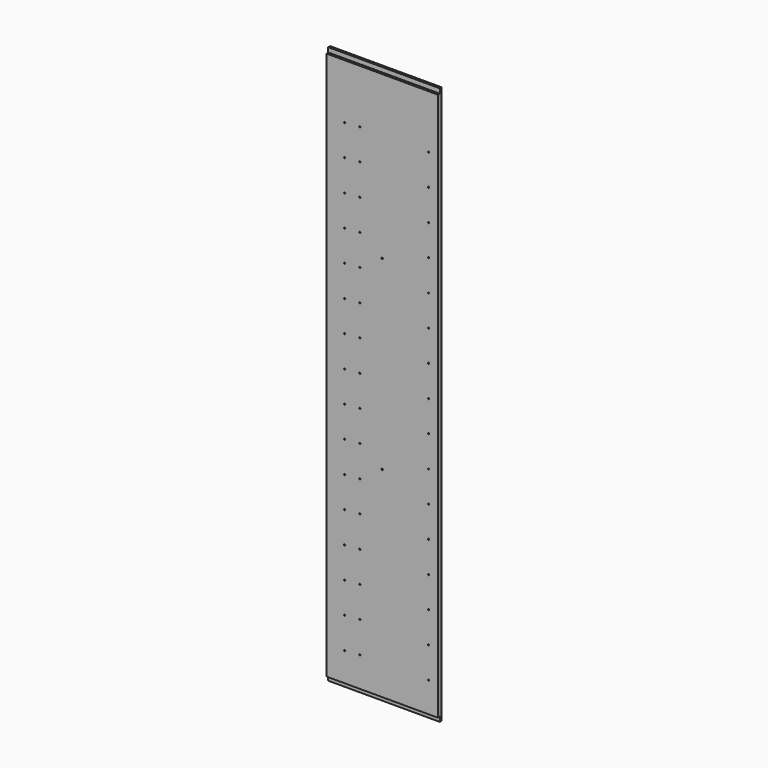
from build123d import *

# Parameters (mm, degrees)
F0_W           = 360
F0_H           = 1750
F1_DEPTH       = 15
F3_D           = 4
F3_DEPTH       = 5
F3_TIP         = 1.2017212381
F5_D           = 5.2
F5_DEPTH       = 15
F5_CBORE_D     = 15.5
F5_CBORE_DEPTH = 3
F5_TIP         = 1.5622376095
F7_W           = 7.5
F7_H           = 15
F8_DEPTH       = 360


# Not quite as in the source:
# - a pattern or mirror of a feature is missing from the dataset's text; its kind, count and spacing are read off the source's solid
# - a feature names something its author has since deleted; it is built from what else it names


with BuildPart() as f1:
    # F0 (on Front) → F1 (new body)
    with BuildSketch(Plane.XZ):
        with Locations((180, 875)):
            Rectangle(F0_W, F0_H)
    extrude(amount=F1_DEPTH)

    # F1_copies: F1 across plane


with BuildPart() as f1_1:
    add(f1.part)
    add(f1.part.mirror(Plane.XY.offset(900)))

    # F3
    with Locations(Plane.XZ.offset(15)):
        with Locations((59, 1308), (108, 812), (330, 1312), (59, 908), (330, 1412), (108, 1412), (59, 1008), (108, 612), (59, 608), (59, 208), (59, 308), (59, 408), (330, 1512), (330, 1212), (59, 808), (108, 1212), (330, 1612), (108, 1512), (108, 1112), (330, 312), (108, 312), (108, 212), (108, 512), (108, 712), (330, 612), (59, 1508), (108, 1312), (330, 912), (59, 1608), (330, 812), (330, 1012), (59, 1408), (330, 212), (108, 1012), (330, 712), (108, 112), (330, 112), (330, 512), (59, 508), (59, 108), (59, 1108), (108, 1612), (59, 1208), (59, 708), (330, 412), (108, 412), (108, 912), (330, 1112)):
            Hole(F3_D / 2, depth=F3_DEPTH)
            with Locations((0, 0, -(F3_DEPTH + F3_TIP / 2))):  # 118° drill point
                Cone(0, F3_D / 2, F3_TIP, mode=Mode.SUBTRACT)

    # F5
    with Locations(Plane(origin=(0, 0, 0), x_dir=(-1, 0, 0), z_dir=(0, 1, 0))):
        with Locations((-180, 1262), (-180, 662)):
            CounterBoreHole(F5_D / 2, F5_CBORE_D / 2, F5_CBORE_DEPTH, depth=F5_DEPTH)
            with Locations((0, 0, -(F5_DEPTH + F5_TIP / 2))):  # 118° drill point
                Cone(0, F5_D / 2, F5_TIP, mode=Mode.SUBTRACT)

    # F7 (on face) → F8 (cut, through all)
    with BuildSketch(Plane(origin=(0, 0, 0), x_dir=(0, -1, 0), z_dir=(-1, 0, 0))):
        with Locations((11.25, 7.5)):
            Rectangle(F7_W, F7_H)
    f8 = extrude(amount=-F8_DEPTH, mode=Mode.SUBTRACT)

    # F8_copies: F8 across plane
    add(f8.mirror(Plane.XY.offset(900)), mode=Mode.SUBTRACT)


solid = f1_1.part
